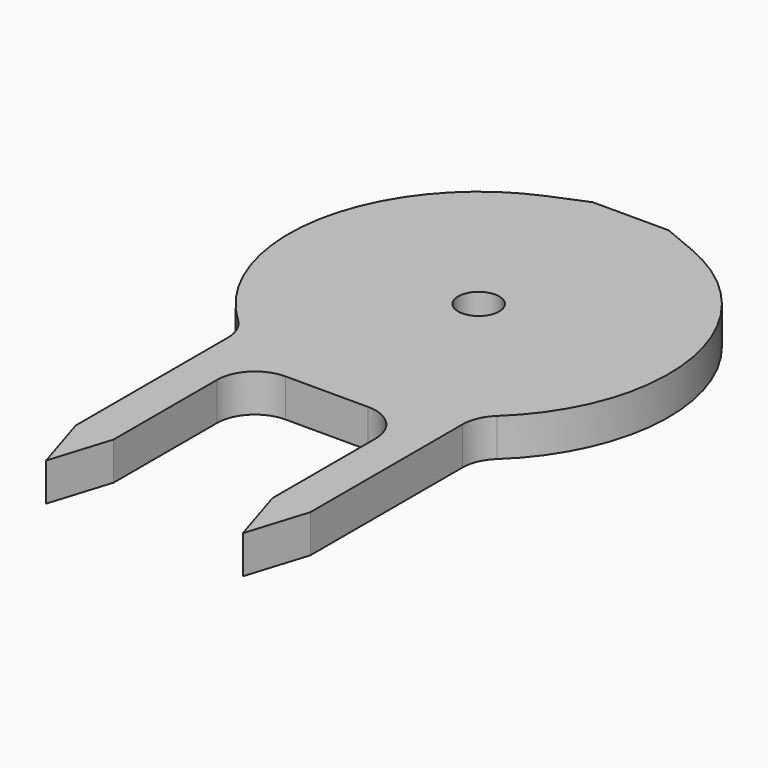
from build123d import *

# Parameters (mm, degrees)
F1_DEPTH = 5
F2_D     = 5.4
F3_W     = 3
F3_H     = 2
F4_DEPTH = 10
F5_R     = 1.49999


# Not quite as in the source:
# - a fillet or chamfer is up to 0.001 mm smaller than in the source, because OpenCascade refuses the exact size


with BuildPart() as f1:
    # F0 (on Top) → F1 (new body)
    with BuildSketch(Plane.XY):
        with BuildLine():
            ThreePointArc((-17.0389572543, 21.7029743907), (-15.8620482104, 20.0392796609), (-15.4467487052, 18.0441552605))
            Line((-15.4467487052, 18.0441552605), (-15.4467487052, -7.0029299584))
            Line((-15.4467487052, -7.0029299584), (-12.9467487052, -15.0029299584))
            Line((-12.9467487052, -15.0029299584), (-10.4467487052, -7.0029299584))
            Line((-10.4467487052, -7.0029299584), (-10.4467487052, 9.9970700416))
            ThreePointArc((-10.4467487052, 9.9970700416), (-8.9822826112, 13.5326039476), (-5.4467487052, 14.9970700416))
            Line((-5.4467487052, 14.9970700416), (0, 14.9970700416))
            Line((0, 14.9970700416), (0, 37.4970700416))
            ThreePointArc((0, 37.4970700416), (-2.5, 39.9970700416), (0, 42.4970700416))
            Line((0, 42.4970700416), (0, 64.9970700416))
            Line((0, 64.9970700416), (-5, 64.9970700416))
            Line((-5, 64.9970700416), (-9.6153846154, 63.0739931186))
            ThreePointArc((-9.6153846154, 63.0739931186), (-24.6069864626, 44.4125221395), (-17.0389572543, 21.7029743907))
        make_face()
        with BuildLine():
            Line((0, 37.4970700416), (0, 42.4970700416))
            ThreePointArc((0, 42.4970700416), (-2.5, 39.9970700416), (0, 37.4970700416))
        make_face()
        with BuildLine():
            Line((5, 64.9970700416), (0, 64.9970700416))
            Line((0, 64.9970700416), (0, 42.4970700416))
            ThreePointArc((0, 42.4970700416), (2.5, 39.9970700416), (0, 37.4970700416))
            Line((0, 37.4970700416), (0, 14.9970700416))
            Line((0, 14.9970700416), (5.4467487052, 14.9970700416))
            ThreePointArc((5.4467487052, 14.9970700416), (8.9822826112, 13.5326039476), (10.4467487052, 9.9970700416))
            Line((10.4467487052, 9.9970700416), (10.4467487052, -7.0029299584))
            Line((10.4467487052, -7.0029299584), (12.9467487052, -15.0029299584))
            Line((12.9467487052, -15.0029299584), (15.4467487052, -7.0029299584))
            Line((15.4467487052, -7.0029299584), (15.4467487052, 18.0441552605))
            ThreePointArc((15.4467487052, 18.0441552605), (15.8620482104, 20.0392796609), (17.0389572543, 21.7029743907))
            ThreePointArc((17.0389572543, 21.7029743907), (24.6069864626, 44.4125221395), (9.6153846154, 63.0739931186))
            Line((9.6153846154, 63.0739931186), (5, 64.9970700416))
        make_face()
        with BuildLine():
            ThreePointArc((0, 37.4970700416), (2.5, 39.9970700416), (0, 42.4970700416))
            Line((0, 42.4970700416), (0, 37.4970700416))
        make_face()
    extrude(amount=F1_DEPTH)

    # F2 (through all)
    with Locations(Plane(origin=(0, 0, 0), x_dir=(1, 0, 0), z_dir=(0, 0, -1))):
        with Locations((0, -39.9970700416)):
            Hole(F2_D / 2)

    # F3 (on face) → F4 (cut)
    with BuildSketch(Plane(origin=(0, 64.9970700416, 0), x_dir=(-1, 0, 0), z_dir=(0, 1, 0))):
        with Locations((0, 2.5)):
            Rectangle(F3_W, F3_H)
    extrude(amount=-F4_DEPTH, mode=Mode.SUBTRACT)

    # F5 (radius 1.5 in the source; OpenCascade refuses exactly that, so slightly less here)
    f5_edges = [f1.edges().sort_by_distance(p)[0] for p in [
        (1.5, 59.99707, 3.5),
        (-1.5, 59.99707, 3.5),
    ]]
    fillet(f5_edges, radius=F5_R)


solid = f1.part
